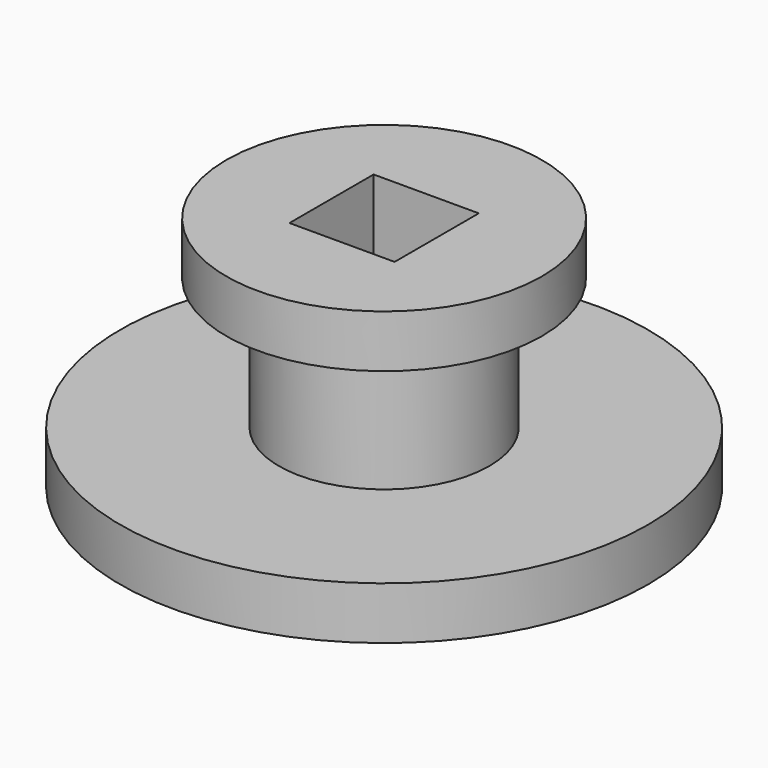
from build123d import *

# Parameters (mm, degrees)
F0_R      = 63.7442234454
F1_DEPTH  = 12.7
F2_R      = 25.4
F3_DEPTH  = 19.05
F4_R      = 9.525
F5_DEPTH  = 50.8
F6_DEPTH  = 12.7
F7_R      = 38.1
F8_DEPTH  = 12.7
F9_W      = 25.4
F9_H      = 25.4
F10_DEPTH = 25.4


with BuildPart() as f1:
    # F0 (on Top) → F1 (new body)
    with BuildSketch(Plane.XY):
        Circle(F0_R)
    extrude(amount=F1_DEPTH)

    # F2 (on face) → F3 (join)
    with BuildSketch(Plane.XY.offset(12.7)):
        Circle(F2_R)
    extrude(amount=F3_DEPTH)

    # F4 (on face) → F5 (cut)
    with BuildSketch(Plane.XY.offset(31.75)):
        Circle(F4_R)
    extrude(amount=-F5_DEPTH, mode=Mode.SUBTRACT)

    # F6 (add): a face of the model
    f6_faces = [f1.faces().sort_by_distance(p)[0] for p in [
        (-24.6815795103, 0, 31.75),
    ]]
    extrude(f6_faces, amount=F6_DEPTH)

    # F7 (on face) → F8 (join)
    with BuildSketch(Plane.XY.offset(44.45)):
        Circle(F7_R)
    extrude(amount=F8_DEPTH)

    # F9 (on face) → F10 (cut)
    with BuildSketch(Plane.XY.offset(57.15)):
        Rectangle(F9_W, F9_H)
    extrude(amount=-F10_DEPTH, mode=Mode.SUBTRACT)


solid = f1.part
